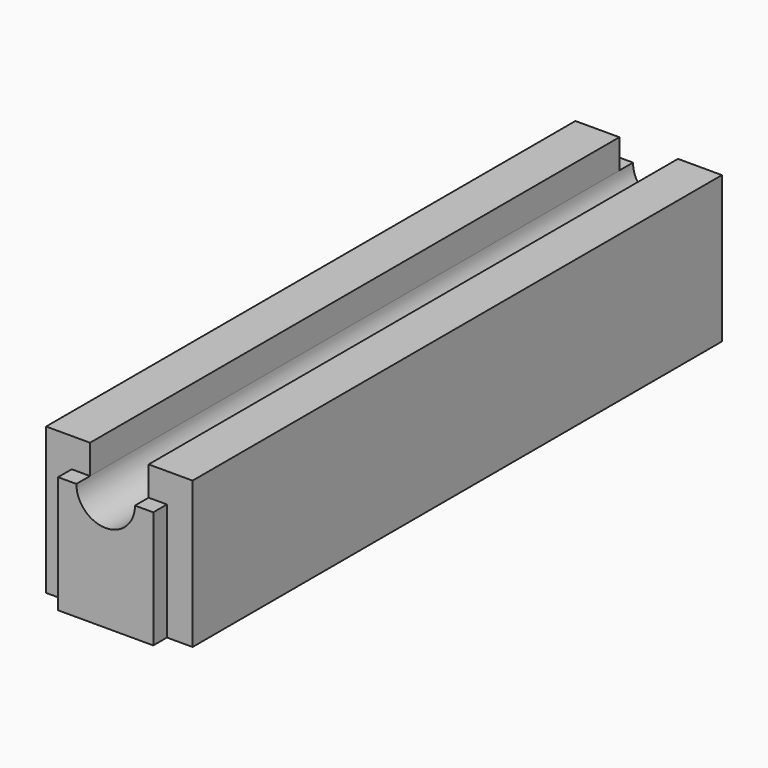
from build123d import *

# Parameters (mm, degrees)
F0_W     = 30
F0_H     = 30
F1_DEPTH = 71.25
F3_DEPTH = 71.251
F4_W     = 5.25
F4_H     = 24
F5_DEPTH = 3.5


# Not quite as in the source:
# - a feature names something its author has since deleted; it is built from what else it names


with BuildPart() as f1:
    # F0 (on Front) → F1 (new body)
    with BuildSketch(Plane.XZ):
        Rectangle(F0_W, F0_H)
    extrude(amount=F1_DEPTH)

    # F2 (on face) → F3 (cut, through all)
    with BuildSketch(Plane.XZ.offset(71.25)):
        with BuildLine():
            Line((6, 9), (6, 15))
            Line((6, 15), (-6, 15))
            Line((-6, 15), (-6, 9))
            ThreePointArc((-6, 9), (0, 3), (6, 9))
        make_face()
    extrude(amount=-F3_DEPTH, mode=Mode.SUBTRACT)

    # F4 (on face) → F5 (cut)
    with BuildSketch(Plane.XZ.offset(71.25)):
        with BuildLine():
            ThreePointArc((-9.75, 9), (-9.2193635213, 12.1726702101), (-7.6852130745, 15))
            Line((-7.6852130745, 15), (-15, 15))
            Line((-15, 15), (-15, 9))
            Line((-15, 9), (-9.75, 9))
        make_face()
        with BuildLine():
            Line((6, 9), (9.75, 9))
            ThreePointArc((9.75, 9), (9.2193635213, 12.1726702101), (7.6852130745, 15))
            Line((7.6852130745, 15), (6, 15))
            Line((6, 15), (6, 9))
        make_face()
        with BuildLine():
            ThreePointArc((7.6852130745, 15), (9.2193635213, 12.1726702101), (9.75, 9))
            Line((9.75, 9), (15, 9))
            Line((15, 9), (15, 15))
            Line((15, 15), (7.6852130745, 15))
        make_face()
        with Locations((-12.375, -3)):
            Rectangle(F4_W, F4_H)
        with Locations((12.375, -3)):
            Rectangle(F4_W, F4_H)
        with BuildLine():
            Line((-6, 15), (-7.6852130745, 15))
            ThreePointArc((-7.6852130745, 15), (-9.2193635213, 12.1726702101), (-9.75, 9))
            Line((-9.75, 9), (-6, 9))
            Line((-6, 9), (-6, 15))
        make_face()
    extrude(amount=-F5_DEPTH, mode=Mode.SUBTRACT)

    # F6: F1 across plane


with BuildPart() as f1_1:
    add(f1.part)
    add(f1.part.mirror(Plane.XZ))


solid = f1_1.part
